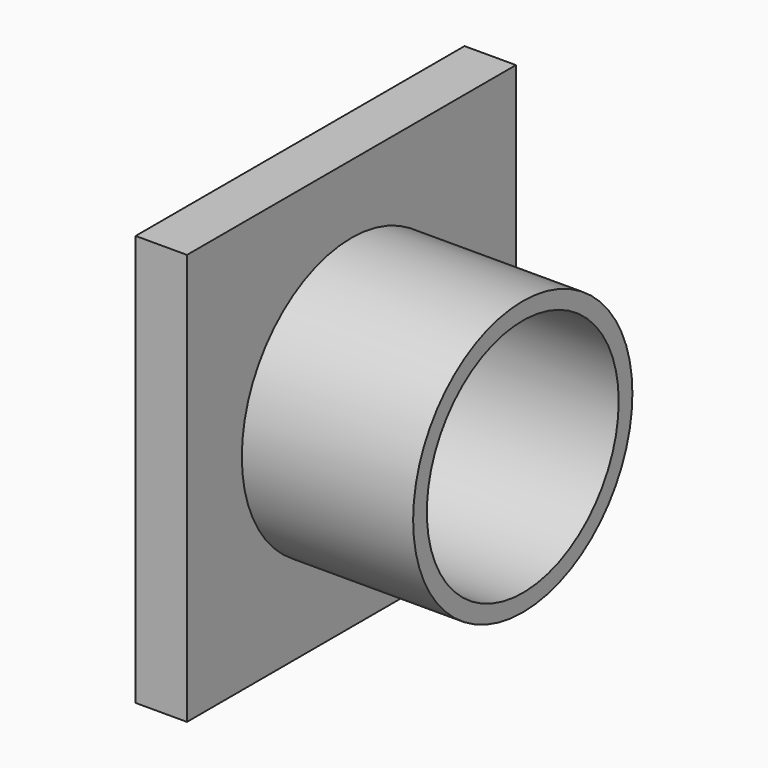
from build123d import *
from build123d import SkipClean  # not in build123d's __all__

# Parameters (mm, degrees)
F0_W     = 152.4
F0_H     = 152.4
F1_DEPTH = 19.05
F2_R     = 44.45
F3_DEPTH = 19.051
F4_R     = 50.8
F4_R_2   = 44.45
F5_DEPTH = 63.5


with BuildPart() as f1:
    # F0 (on Right) → F1 (new body)
    with BuildSketch(Plane.YZ):
        Rectangle(F0_W, F0_H)
    extrude(amount=F1_DEPTH)

    # F2 (on face) → F3 (cut, through all)
    with BuildSketch(Plane(origin=(0, 0, 0), x_dir=(0, -1, 0), z_dir=(-1, 0, 0))):
        Circle(F2_R)
    extrude(amount=-F3_DEPTH, mode=Mode.SUBTRACT)

    # F4 (on face) → F5 (join)
    with BuildSketch(Plane.YZ.offset(19.05)):
        Circle(F4_R)
        Circle(F4_R_2, mode=Mode.SUBTRACT)
    with SkipClean():  # cleaning this boolean's faces spoils the solid; the shape is the same uncleaned
        extrude(amount=F5_DEPTH)


solid = f1.part
